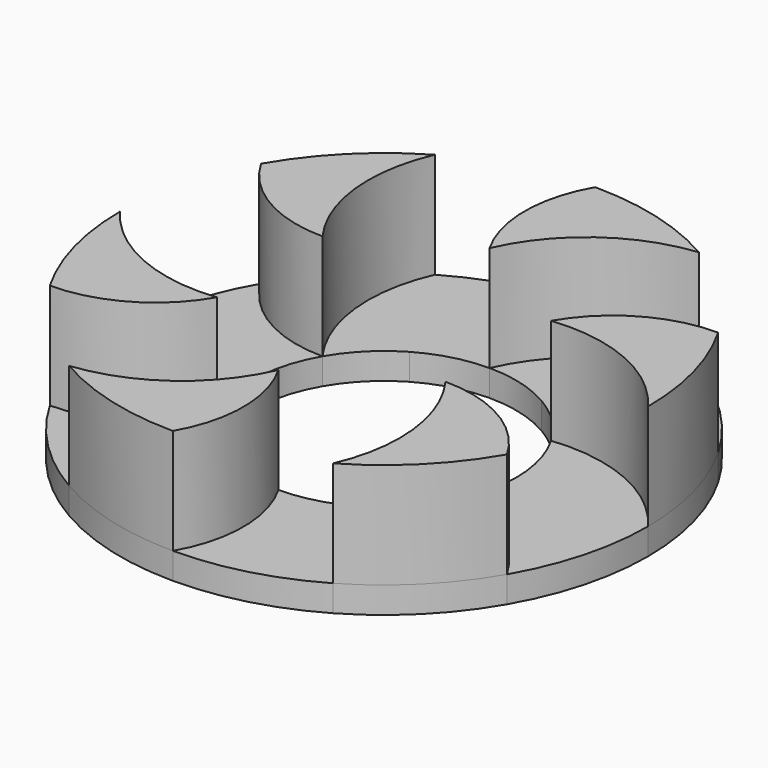
from build123d import *

# Parameters (mm, degrees)
F1_DEPTH = 10
F2_DEPTH = 2.5


with BuildPart() as f1:
    # F0 (on Top) → F1 (new body)
    with BuildSketch(Plane.XY):
        with BuildLine():
            ThreePointArc((10.8253175473, 6.25), (18.75, 5.0240473581), (25, 0))
            ThreePointArc((25, 0), (24.1481456572, 6.4704761276), (21.6506350946, 12.5))
            ThreePointArc((21.6506350946, 12.5), (15.4006350946, 10.8253175473), (10.8253175473, 6.25))
        make_face()
    extrude(amount=F1_DEPTH)


with BuildPart() as f1b:
    # F0 (on Top) → F1, piece 2 (new body)
    with BuildSketch(Plane.XY):
        with BuildLine():
            ThreePointArc((12.5, -21.6506350946), (17.6776695297, -17.6776695297), (21.6506350946, -12.5))
            ThreePointArc((21.6506350946, -12.5), (17.0753175473, -7.9246824527), (10.8253175473, -6.25))
            ThreePointArc((10.8253175473, -6.25), (13.7259526419, -13.7259526419), (12.5, -21.6506350946))
        make_face()
    extrude(amount=F1_DEPTH)


with BuildPart() as f1c:
    # F0 (on Top) → F1, piece 3 (new body)
    with BuildSketch(Plane.XY):
        with BuildLine():
            ThreePointArc((0, 12.5), (5.0240473581, 18.75), (12.5, 21.6506350946))
            ThreePointArc((12.5, 21.6506350946), (6.4704761276, 24.1481456572), (0, 25))
            ThreePointArc((0, 25), (-1.6746824527, 18.75), (0, 12.5))
        make_face()
    extrude(amount=F1_DEPTH)


with BuildPart() as f1d:
    # F0 (on Top) → F1, piece 4 (new body)
    with BuildSketch(Plane.XY):
        with BuildLine():
            ThreePointArc((-12.5, -21.6506350946), (-6.4704761276, -24.1481456572), (0, -25))
            ThreePointArc((0, -25), (1.6746824527, -18.75), (0, -12.5))
            ThreePointArc((0, -12.5), (-5.0240473581, -18.75), (-12.5, -21.6506350946))
        make_face()
    extrude(amount=F1_DEPTH)


with BuildPart() as f1e:
    # F0 (on Top) → F1, piece 5 (new body)
    with BuildSketch(Plane.XY):
        with BuildLine():
            ThreePointArc((-21.6506350946, 12.5), (-17.0753175473, 7.9246824527), (-10.8253175473, 6.25))
            ThreePointArc((-10.8253175473, 6.25), (-13.7259526419, 13.7259526419), (-12.5, 21.6506350946))
            ThreePointArc((-12.5, 21.6506350946), (-17.6776695297, 17.6776695297), (-21.6506350946, 12.5))
        make_face()
    extrude(amount=F1_DEPTH)


with BuildPart() as f1f:
    # F0 (on Top) → F1, piece 6 (new body)
    with BuildSketch(Plane.XY):
        with BuildLine():
            ThreePointArc((-21.6506350946, -12.5), (-15.4006350946, -10.8253175473), (-10.8253175473, -6.25))
            ThreePointArc((-10.8253175473, -6.25), (-18.75, -5.0240473581), (-25, 0))
            ThreePointArc((-25, 0), (-24.1481456572, -6.4704761276), (-21.6506350946, -12.5))
        make_face()
    extrude(amount=F1_DEPTH)


with BuildPart() as f2:
    # F0 (on Top) → F2 (new body)
    with BuildSketch(Plane.XY):
        with BuildLine():
            ThreePointArc((10.8253175473, 6.25), (18.75, 5.0240473581), (25, 0))
            ThreePointArc((25, 0), (24.1481456572, 6.4704761276), (21.6506350946, 12.5))
            ThreePointArc((21.6506350946, 12.5), (15.4006350946, 10.8253175473), (10.8253175473, 6.25))
        make_face()
        with BuildLine():
            ThreePointArc((21.6506350946, -12.5), (24.1481456572, -6.4704761276), (25, 0))
            Line((25, 0), (12.5, 0))
            ThreePointArc((12.5, 0), (18.75, -5.0240473581), (21.6506350946, -12.5))
        make_face()
        with BuildLine():
            Line((12.5, 0), (25, 0))
            ThreePointArc((25, 0), (18.75, 5.0240473581), (10.8253175473, 6.25))
            ThreePointArc((10.8253175473, 6.25), (12.0740728286, 3.2352380638), (12.5, 0))
        make_face()
        with BuildLine():
            ThreePointArc((6.25, 10.8253175473), (13.7259526419, 13.7259526419), (21.6506350946, 12.5))
            ThreePointArc((21.6506350946, 12.5), (17.6776695297, 17.6776695297), (12.5, 21.6506350946))
            Line((12.5, 21.6506350946), (6.25, 10.8253175473))
        make_face()
        with BuildLine():
            ThreePointArc((10.8253175473, 6.25), (15.4006350946, 10.8253175473), (21.6506350946, 12.5))
            ThreePointArc((21.6506350946, 12.5), (13.7259526419, 13.7259526419), (6.25, 10.8253175473))
            ThreePointArc((6.25, 10.8253175473), (8.8388347648, 8.8388347648), (10.8253175473, 6.25))
        make_face()
        with BuildLine():
            ThreePointArc((10.8253175473, -6.25), (17.0753175473, -7.9246824527), (21.6506350946, -12.5))
            ThreePointArc((21.6506350946, -12.5), (18.75, -5.0240473581), (12.5, 0))
            ThreePointArc((12.5, 0), (12.0740728286, -3.2352380638), (10.8253175473, -6.25))
        make_face()
        with BuildLine():
            ThreePointArc((12.5, -21.6506350946), (17.6776695297, -17.6776695297), (21.6506350946, -12.5))
            ThreePointArc((21.6506350946, -12.5), (17.0753175473, -7.9246824527), (10.8253175473, -6.25))
            ThreePointArc((10.8253175473, -6.25), (13.7259526419, -13.7259526419), (12.5, -21.6506350946))
        make_face()
        with BuildLine():
            ThreePointArc((0, 12.5), (5.0240473581, 18.75), (12.5, 21.6506350946))
            ThreePointArc((12.5, 21.6506350946), (6.4704761276, 24.1481456572), (0, 25))
            ThreePointArc((0, 25), (-1.6746824527, 18.75), (0, 12.5))
        make_face()
        with BuildLine():
            Line((6.25, 10.8253175473), (12.5, 21.6506350946))
            ThreePointArc((12.5, 21.6506350946), (5.0240473581, 18.75), (0, 12.5))
            ThreePointArc((0, 12.5), (3.2352380638, 12.0740728286), (6.25, 10.8253175473))
        make_face()
        with BuildLine():
            ThreePointArc((0, -25), (6.4704761276, -24.1481456572), (12.5, -21.6506350946))
            Line((12.5, -21.6506350946), (6.25, -10.8253175473))
            ThreePointArc((6.25, -10.8253175473), (5.0240473581, -18.75), (0, -25))
        make_face()
        with BuildLine():
            Line((6.25, -10.8253175473), (12.5, -21.6506350946))
            ThreePointArc((12.5, -21.6506350946), (13.7259526419, -13.7259526419), (10.8253175473, -6.25))
            ThreePointArc((10.8253175473, -6.25), (8.8388347648, -8.8388347648), (6.25, -10.8253175473))
        make_face()
        with BuildLine():
            ThreePointArc((-6.25, 10.8253175473), (-5.0240473581, 18.75), (0, 25))
            ThreePointArc((0, 25), (-6.4704761276, 24.1481456572), (-12.5, 21.6506350946))
            Line((-12.5, 21.6506350946), (-6.25, 10.8253175473))
        make_face()
        with BuildLine():
            ThreePointArc((0, 12.5), (-1.6746824527, 18.75), (0, 25))
            ThreePointArc((0, 25), (-5.0240473581, 18.75), (-6.25, 10.8253175473))
            ThreePointArc((-6.25, 10.8253175473), (-3.2352380638, 12.0740728286), (0, 12.5))
        make_face()
        with BuildLine():
            ThreePointArc((0, -12.5), (1.6746824527, -18.75), (0, -25))
            ThreePointArc((0, -25), (5.0240473581, -18.75), (6.25, -10.8253175473))
            ThreePointArc((6.25, -10.8253175473), (3.2352380638, -12.0740728286), (0, -12.5))
        make_face()
        with BuildLine():
            ThreePointArc((-12.5, -21.6506350946), (-6.4704761276, -24.1481456572), (0, -25))
            ThreePointArc((0, -25), (1.6746824527, -18.75), (0, -12.5))
            ThreePointArc((0, -12.5), (-5.0240473581, -18.75), (-12.5, -21.6506350946))
        make_face()
        with BuildLine():
            ThreePointArc((-12.5, 21.6506350946), (-13.7259526419, 13.7259526419), (-10.8253175473, 6.25))
            ThreePointArc((-10.8253175473, 6.25), (-8.8388347648, 8.8388347648), (-6.25, 10.8253175473))
            Line((-6.25, 10.8253175473), (-12.5, 21.6506350946))
        make_face()
        with BuildLine():
            ThreePointArc((-21.6506350946, 12.5), (-17.0753175473, 7.9246824527), (-10.8253175473, 6.25))
            ThreePointArc((-10.8253175473, 6.25), (-13.7259526419, 13.7259526419), (-12.5, 21.6506350946))
            ThreePointArc((-12.5, 21.6506350946), (-17.6776695297, 17.6776695297), (-21.6506350946, 12.5))
        make_face()
        with BuildLine():
            ThreePointArc((-12.5, 0), (-12.0740728286, 3.2352380638), (-10.8253175473, 6.25))
            ThreePointArc((-10.8253175473, 6.25), (-17.0753175473, 7.9246824527), (-21.6506350946, 12.5))
            ThreePointArc((-21.6506350946, 12.5), (-18.75, 5.0240473581), (-12.5, 0))
        make_face()
        with BuildLine():
            ThreePointArc((-25, 0), (-18.75, -5.0240473581), (-10.8253175473, -6.25))
            ThreePointArc((-10.8253175473, -6.25), (-12.0740728286, -3.2352380638), (-12.5, 0))
            Line((-12.5, 0), (-25, 0))
        make_face()
        with BuildLine():
            ThreePointArc((-21.6506350946, -12.5), (-15.4006350946, -10.8253175473), (-10.8253175473, -6.25))
            ThreePointArc((-10.8253175473, -6.25), (-18.75, -5.0240473581), (-25, 0))
            ThreePointArc((-25, 0), (-24.1481456572, -6.4704761276), (-21.6506350946, -12.5))
        make_face()
        with BuildLine():
            ThreePointArc((-6.25, -10.8253175473), (-8.8388347648, -8.8388347648), (-10.8253175473, -6.25))
            ThreePointArc((-10.8253175473, -6.25), (-15.4006350946, -10.8253175473), (-21.6506350946, -12.5))
            ThreePointArc((-21.6506350946, -12.5), (-13.7259526419, -13.7259526419), (-6.25, -10.8253175473))
        make_face()
        with BuildLine():
            ThreePointArc((-12.5, -21.6506350946), (-5.0240473581, -18.75), (0, -12.5))
            ThreePointArc((0, -12.5), (-3.2352380638, -12.0740728286), (-6.25, -10.8253175473))
            Line((-6.25, -10.8253175473), (-12.5, -21.6506350946))
        make_face()
        with BuildLine():
            ThreePointArc((-21.6506350946, -12.5), (-17.6776695297, -17.6776695297), (-12.5, -21.6506350946))
            Line((-12.5, -21.6506350946), (-6.25, -10.8253175473))
            ThreePointArc((-6.25, -10.8253175473), (-13.7259526419, -13.7259526419), (-21.6506350946, -12.5))
        make_face()
        with BuildLine():
            Line((-25, 0), (-12.5, 0))
            ThreePointArc((-12.5, 0), (-18.75, 5.0240473581), (-21.6506350946, 12.5))
            ThreePointArc((-21.6506350946, 12.5), (-24.1481456572, 6.4704761276), (-25, 0))
        make_face()
    extrude(amount=-F2_DEPTH)


solid = Compound([f1.part, f1b.part, f1c.part, f1d.part, f1e.part, f1f.part, f2.part])
